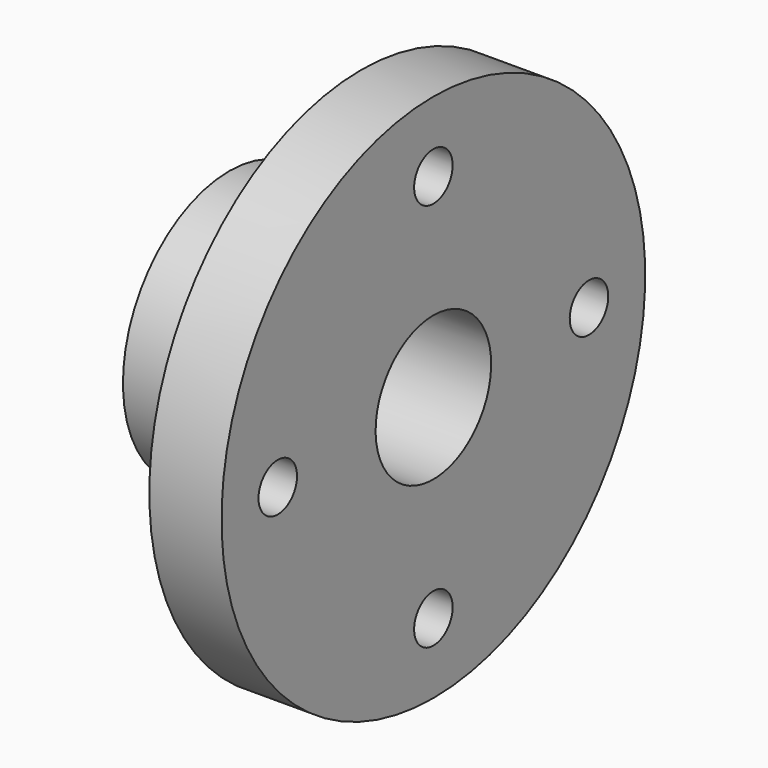
from build123d import *

# Parameters (mm, degrees)
F2_R            = 6.35
F3_DEPTH        = 25.4
F3_COPIES_COUNT = 4


# Not quite as in the source:
# - a pattern or mirror of a feature is missing from the dataset's text; its kind, count and spacing are read off the source's solid


with BuildPart() as f1:
    # F0 (on Front) → F1 (revolve)
    with BuildSketch(Plane.XZ):
        Polygon((-53.848, 19.05), (0, 19.05), (0, 69.85), (-19.05, 69.85), (-19.05, 35.052), (-53.848, 35.052), align=None)
    revolve(axis=Axis((-30.7231917977, 0, 0), (-1, 0, 0)))

    # F2 (on Right) → F3 (cut)
    with BuildSketch(Plane.YZ):
        with Locations((0, 51.308)):
            Circle(F2_R)
    f3 = extrude(amount=-F3_DEPTH, mode=Mode.SUBTRACT)

    # F3_copies: F3 ×4 about axis
    f3_copies_axis = Axis((0, 0, 0), (1, 0, 0))
    for i in range(1, F3_COPIES_COUNT):
        add(f3.rotate(f3_copies_axis, i * 360 / F3_COPIES_COUNT), mode=Mode.SUBTRACT)


solid = f1.part
